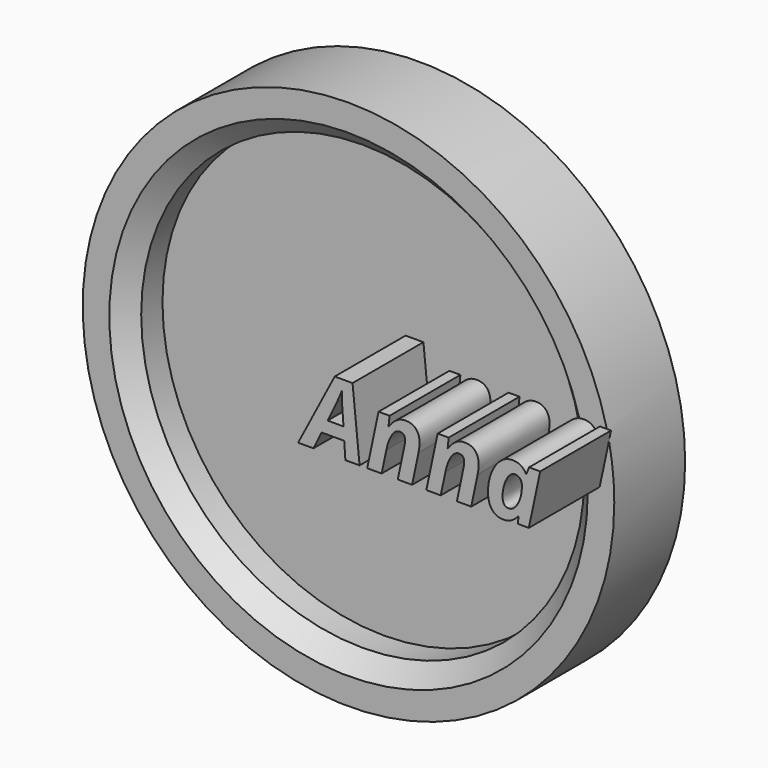
from build123d import *

# Parameters (mm, degrees)
F0_R         = 76.2
F1_DEPTH     = 25.4
F3_T         = -12.7
F4_SIZE      = 5.08
F5_TEXT_SIZE = 28.0593948749
F6_DEPTH     = 25.4


# Not quite as in the source:
# - Text() gives the source's letters only with a copy of the font that has no kerning and outlines rounded to 1/6400 em; it was checked with that copy


with BuildPart() as f1:
    # F0 (on Front) → F1 (new body)
    with BuildSketch(Plane.XZ):
        Circle(F0_R)
    extrude(amount=F1_DEPTH)

    # F3
    f3_openings = [f1.faces().sort_by_distance(p)[0] for p in [
        (0, -25.4, 0),
    ]]
    offset(amount=F3_T, openings=f3_openings)

    # F4
    f4_edges = [f1.edges().sort_by_distance(p)[0] for p in [
        (-63.5, -25.4, 0),
    ]]
    chamfer(f4_edges, length=F4_SIZE)

    # F5 (on face) → F6 (join)
    with BuildSketch(Plane.XZ.offset(25.4)):
        with Locations((7.5582005084, 2.5878595188)):
            Text('Anna', F5_TEXT_SIZE, font='Open Sans', font_style=FontStyle.BOLDITALIC, text_align=(TextAlign.LEFT, TextAlign.BOTTOM))
    extrude(amount=F6_DEPTH)


solid = f1.part
